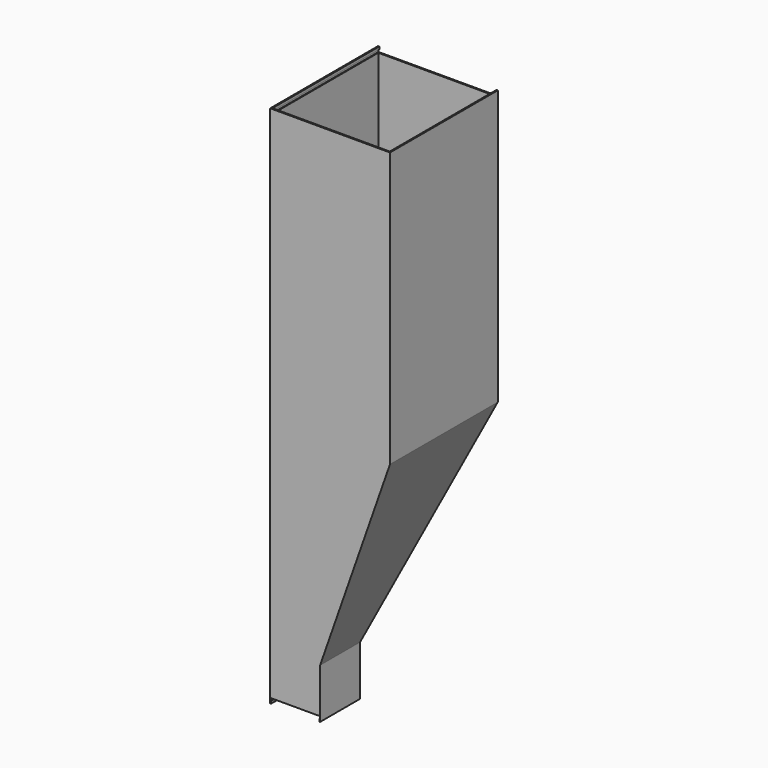
from build123d import *

# Parameters (mm, degrees)
F0_W        = 100
F0_H        = 100
F1_DEPTH    = 135
F3_DEPTH    = 240
F4_T        = 2.5
F4_T3_DEPTH = 105
F4_T5_DEPTH = 105
F6_DEPTH    = 98.5
F7_W        = 235
F7_H        = 5
F8_DEPTH    = 2.5
F9_DEPTH    = 269


# Not quite as in the source:
# - a shell that OpenCascade refuses in one call is made with other operations: the cavity is built on its own and cut out


with BuildPart() as f1:
    # F0 (on Front) → F1 (new body, symmetric)
    with BuildSketch(Plane.XZ):
        Polygon((0, 500), (0, 100), (100, 100), (240, 500), (240, 1050), (0, 1050), align=None)
        with Locations((50, 50)):
            Rectangle(F0_W, F0_H)
    extrude(amount=F1_DEPTH, both=True)

    # F2 (on face) → F3 (cut)
    with BuildSketch(Plane.YZ.offset(240)):
        Polygon((135, 0), (135, 500), (-35, 100), (-35, 0), align=None)
    extrude(amount=-F3_DEPTH, mode=Mode.SUBTRACT)

    # F4: shell of thickness 2.5, made by hand


with BuildPart() as f4_core1:
    # F4_t2: copy of F1
    add(f1.part)

    # the walls: a layer under each face that stays
    f4_faces = [f4_core1.faces().sort_by_distance(p)[0] for p in [
        (0, 0, 525),
        (120, -135, 525),
        (100, -85, 50),
        (50, -35, 50),
        (120, 50, 300),
        (120, 135, 775),
        (170, 0, 300),
        (240, 0, 775),
    ]]
    thicken(f4_faces, amount=-F4_T, mode=Mode.SUBTRACT)

    # F4_s4 → F4_t3 (cut)
    with BuildSketch(Plane.XZ.offset(32.5)):
        Polygon((100.0485964589, 99.9917412394), (97.5, 100), (97.5, 100.4248643216), (97.6403541091, 100.8258760618), align=None)
    extrude(amount=F4_T3_DEPTH, mode=Mode.SUBTRACT)

    # F4_s6 → F4_t5 (cut)
    with BuildSketch(Plane.YZ.offset(-2.5)):
        Polygon((-34.951991727, 99.990221484), (-37.5, 100), (-37.5, 100.5092099447), (-37.3008272961, 100.9778516009), align=None)
    extrude(amount=F4_T5_DEPTH, mode=Mode.SUBTRACT)


with BuildPart() as f1_1:
    add(f1.part)

    # what is left inside the walls is the cavity
    f4_cavity = [f4_core1.part.solids().sort_by_distance(p)[0] for p in [
        (2.525, 44.166667, 525),
    ]]
    add(f4_cavity, mode=Mode.SUBTRACT)

    # F5 (on face) → F6 (cut)
    with BuildSketch(Plane.XZ.offset(135)):
        Polygon((1.5, 5), (1.5, 0), (98.5, 0), (98.5, 5), (99.5, 5), (99.5, 10), (0.5, 10), (0.5, 5), align=None)
    extrude(amount=-F6_DEPTH, mode=Mode.SUBTRACT)

    # F7 (on face) → F8 (cut)
    with BuildSketch(Plane(origin=(0, 135, 0), x_dir=(-1, 0, 0), z_dir=(0, 1, 0))):
        with Locations((-120, 1047.5)):
            Rectangle(F7_W, F7_H)
    extrude(amount=-F8_DEPTH, mode=Mode.SUBTRACT)

    # F7 (on face) → F9 (cut)
    with BuildSketch(Plane(origin=(0, 135, 0), x_dir=(-1, 0, 0), z_dir=(0, 1, 0))):
        Polygon((-2.5, 1045), (-237.5, 1045), (-239, 1045), (-239, 1040), (-1, 1040), (-1, 1045), align=None)
    extrude(amount=-F9_DEPTH, mode=Mode.SUBTRACT)


solid = f1_1.part
